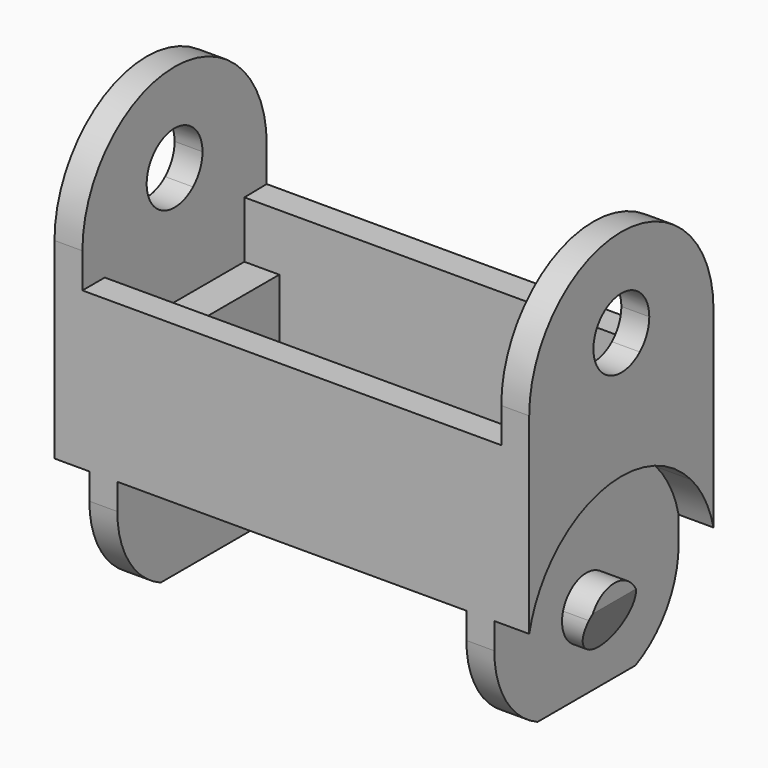
from build123d import *

# Parameters (mm, degrees)
F2_DEPTH = 1.6
F3_DEPTH = 2
F4_DEPTH = 0.4
F5_DEPTH = 11.6
F6_DEPTH = 2
F7_DEPTH = 1.6
F9_DEPTH = 25


# Not quite as in the source:
# - a feature names something its author has since deleted; it is built from what else it names


with BuildPart() as f2:
    # F1 (on offset) → F2 (new body)
    with BuildSketch(Plane.YZ.offset(11.6)):
        with BuildLine():
            Line((-0.1658547654, -17.9765316878), (-0.1658547654, -20.645576419))
            ThreePointArc((-0.1658547654, -20.645576419), (4.8341452346, -18.4390658066), (9.8341452346, -20.645576419))
            Line((9.8341452346, -20.645576419), (9.8341452346, -17.9765316878))
            Line((9.8341452346, -17.9765316878), (-0.1658547654, -17.9765316878))
        make_face()
        with BuildLine():
            Line((-0.1658547654, -23.7073743102), (-1.7658547654, -23.7073743102))
            Line((-1.7658547654, -23.7073743102), (-1.7658547654, -25.2073743102))
            Line((-1.7658547654, -25.2073743102), (-0.1658547654, -25.2073743102))
            Line((-0.1658547654, -25.2073743102), (3.1570942515, -25.2073743102))
            ThreePointArc((3.1570942515, -25.2073743102), (4.8341452346, -23.9573743102), (6.5111962178, -25.2073743102))
            Line((6.5111962178, -25.2073743102), (9.8341452346, -25.2073743102))
            Line((9.8341452346, -25.2073743102), (11.4341452346, -25.2073743102))
            Line((11.4341452346, -25.2073743102), (11.4341452346, -23.7073743102))
            Line((11.4341452346, -23.7073743102), (9.8341452346, -23.7073743102))
            Line((9.8341452346, -23.7073743102), (9.8341452346, -20.645576419))
            ThreePointArc((9.8341452346, -20.645576419), (4.8341452346, -18.4390658066), (-0.1658547654, -20.645576419))
            Line((-0.1658547654, -20.645576419), (-0.1658547654, -23.7073743102))
        make_face()
        with BuildLine():
            Line((-0.1658547654, -25.2073743102), (-1.7658547654, -25.2073743102))
            ThreePointArc((-1.7658547654, -25.2073743102), (-0.9246460766, -28.0854161792), (1.3341452346, -30.0573743102))
            Line((1.3341452346, -30.0573743102), (8.3341452346, -30.0573743102))
            ThreePointArc((8.3341452346, -30.0573743102), (10.5929365459, -28.0854161792), (11.4341452346, -25.2073743102))
            Line((11.4341452346, -25.2073743102), (9.8341452346, -25.2073743102))
            Line((9.8341452346, -25.2073743102), (6.5111962178, -25.2073743102))
            ThreePointArc((6.5111962178, -25.2073743102), (6.5658119492, -25.4547275414), (6.5841452346, -25.7073743102))
            ThreePointArc((6.5841452346, -25.7073743102), (4.5814984659, -27.4390410247), (3.1570942515, -25.2073743102))
            Line((3.1570942515, -25.2073743102), (-0.1658547654, -25.2073743102))
        make_face()
        with BuildLine():
            Line((6.5111962178, -25.2073743102), (3.1570942515, -25.2073743102))
            ThreePointArc((3.1570942515, -25.2073743102), (4.5814984659, -27.4390410247), (6.5841452346, -25.7073743102))
            ThreePointArc((6.5841452346, -25.7073743102), (6.5658119492, -25.4547275414), (6.5111962178, -25.2073743102))
        make_face()
        with BuildLine():
            ThreePointArc((6.5111962178, -25.2073743102), (4.8341452346, -23.9573743102), (3.1570942515, -25.2073743102))
            Line((3.1570942515, -25.2073743102), (6.5111962178, -25.2073743102))
        make_face()
        with BuildLine():
            Line((9.8341452346, -23.7073743102), (11.4341452346, -23.7073743102))
            ThreePointArc((11.4341452346, -23.7073743102), (10.8327827117, -22.0726736198), (9.8341452346, -20.645576419))
            Line((9.8341452346, -20.645576419), (9.8341452346, -23.7073743102))
        make_face()
        with BuildLine():
            ThreePointArc((-0.1658547654, -20.645576419), (-1.1644922425, -22.0726736198), (-1.7658547654, -23.7073743102))
            Line((-1.7658547654, -23.7073743102), (-0.1658547654, -23.7073743102))
            Line((-0.1658547654, -23.7073743102), (-0.1658547654, -20.645576419))
        make_face()
    extrude(amount=-F2_DEPTH)

    # F1 (on offset) → F3 (join)
    with BuildSketch(Plane.YZ.offset(11.6)):
        with BuildLine():
            Line((-0.1658547654, -12.7073743102), (-1.7658547654, -12.7073743102))
            Line((-1.7658547654, -12.7073743102), (-1.7658547654, -14.7073743102))
            Line((-1.7658547654, -14.7073743102), (-0.1658547654, -14.7073743102))
            Line((-0.1658547654, -14.7073743102), (-0.1658547654, -17.9765316878))
            Line((-0.1658547654, -17.9765316878), (9.8341452346, -17.9765316878))
            Line((9.8341452346, -17.9765316878), (9.8341452346, -14.7278557842))
            Line((9.8341452346, -14.7278557842), (11.4341452346, -14.7073743102))
            Line((11.4341452346, -14.7073743102), (11.4341452346, -12.7073743102))
            Line((11.4341452346, -12.7073743102), (9.8341452346, -12.7073743102))
            Line((9.8341452346, -12.7073743102), (6.1570208902, -12.7073743102))
            ThreePointArc((6.1570208902, -12.7073743102), (4.8341452346, -13.2073743102), (3.5112695791, -12.7073743102))
            Line((3.5112695791, -12.7073743102), (-0.1658547654, -12.7073743102))
        make_face()
        with BuildLine():
            ThreePointArc((11.4341452346, -12.7073743102), (4.8341452346, -6.1073743102), (-1.7658547654, -12.7073743102))
            Line((-1.7658547654, -12.7073743102), (-0.1658547654, -12.7073743102))
            Line((-0.1658547654, -12.7073743102), (3.5112695791, -12.7073743102))
            ThreePointArc((3.5112695791, -12.7073743102), (4.0112695791, -9.3844986547), (6.8341452346, -11.2073743102))
            ThreePointArc((6.8341452346, -11.2073743102), (6.6570208902, -12.0302499657), (6.1570208902, -12.7073743102))
            Line((6.1570208902, -12.7073743102), (9.8341452346, -12.7073743102))
            Line((9.8341452346, -12.7073743102), (11.4341452346, -12.7073743102))
        make_face()
        with BuildLine():
            Line((-0.1658547654, -17.9765316878), (-0.1658547654, -20.645576419))
            ThreePointArc((-0.1658547654, -20.645576419), (4.8341452346, -18.4390658066), (9.8341452346, -20.645576419))
            Line((9.8341452346, -20.645576419), (9.8341452346, -17.9765316878))
            Line((9.8341452346, -17.9765316878), (-0.1658547654, -17.9765316878))
        make_face()
    extrude(amount=F3_DEPTH)

    # F1 (on offset) → F4 (cut)
    with BuildSketch(Plane.YZ.offset(11.6)):
        with BuildLine():
            Line((-0.1658547654, -12.7073743102), (-1.7658547654, -12.7073743102))
            Line((-1.7658547654, -12.7073743102), (-1.7658547654, -14.7073743102))
            Line((-1.7658547654, -14.7073743102), (-0.1658547654, -14.7073743102))
            Line((-0.1658547654, -14.7073743102), (-0.1658547654, -17.9765316878))
            Line((-0.1658547654, -17.9765316878), (9.8341452346, -17.9765316878))
            Line((9.8341452346, -17.9765316878), (9.8341452346, -14.7278557842))
            Line((9.8341452346, -14.7278557842), (11.4341452346, -14.7073743102))
            Line((11.4341452346, -14.7073743102), (11.4341452346, -12.7073743102))
            Line((11.4341452346, -12.7073743102), (9.8341452346, -12.7073743102))
            Line((9.8341452346, -12.7073743102), (6.1570208902, -12.7073743102))
            ThreePointArc((6.1570208902, -12.7073743102), (4.8341452346, -13.2073743102), (3.5112695791, -12.7073743102))
            Line((3.5112695791, -12.7073743102), (-0.1658547654, -12.7073743102))
        make_face()
        with BuildLine():
            ThreePointArc((11.4341452346, -12.7073743102), (4.8341452346, -6.1073743102), (-1.7658547654, -12.7073743102))
            Line((-1.7658547654, -12.7073743102), (-0.1658547654, -12.7073743102))
            Line((-0.1658547654, -12.7073743102), (3.5112695791, -12.7073743102))
            ThreePointArc((3.5112695791, -12.7073743102), (4.0112695791, -9.3844986547), (6.8341452346, -11.2073743102))
            ThreePointArc((6.8341452346, -11.2073743102), (6.6570208902, -12.0302499657), (6.1570208902, -12.7073743102))
            Line((6.1570208902, -12.7073743102), (9.8341452346, -12.7073743102))
            Line((9.8341452346, -12.7073743102), (11.4341452346, -12.7073743102))
        make_face()
    extrude(amount=F4_DEPTH, mode=Mode.SUBTRACT)



with BuildPart() as f5:
    # F1 (on offset) → F5 (new body)
    with BuildSketch(Plane.YZ.offset(11.6)):
        with BuildLine():
            Line((11.4341452346, -23.7073743102), (11.4341452346, -14.7073743102))
            Line((11.4341452346, -14.7073743102), (9.8341452346, -14.7278557842))
            Line((9.8341452346, -14.7278557842), (9.8341452346, -17.9765316878))
            Line((9.8341452346, -17.9765316878), (9.8341452346, -20.645576419))
            ThreePointArc((9.8341452346, -20.645576419), (10.8327827117, -22.0726736198), (11.4341452346, -23.7073743102))
        make_face()
        with BuildLine():
            Line((9.8341452346, -23.7073743102), (11.4341452346, -23.7073743102))
            ThreePointArc((11.4341452346, -23.7073743102), (10.8327827117, -22.0726736198), (9.8341452346, -20.645576419))
            Line((9.8341452346, -20.645576419), (9.8341452346, -23.7073743102))
        make_face()
    extrude(amount=-F5_DEPTH)


with BuildPart() as f5b:
    # F1 (on offset) → F5, piece 2 (new body)
    with BuildSketch(Plane.YZ.offset(11.6)):
        with BuildLine():
            Line((-0.1658547654, -14.7073743102), (-1.7658547654, -14.7073743102))
            Line((-1.7658547654, -14.7073743102), (-1.7658547654, -23.7073743102))
            ThreePointArc((-1.7658547654, -23.7073743102), (-1.1644922425, -22.0726736198), (-0.1658547654, -20.645576419))
            Line((-0.1658547654, -20.645576419), (-0.1658547654, -17.9765316878))
            Line((-0.1658547654, -17.9765316878), (-0.1658547654, -14.7073743102))
        make_face()
        with BuildLine():
            ThreePointArc((-0.1658547654, -20.645576419), (-1.1644922425, -22.0726736198), (-1.7658547654, -23.7073743102))
            Line((-1.7658547654, -23.7073743102), (-0.1658547654, -23.7073743102))
            Line((-0.1658547654, -23.7073743102), (-0.1658547654, -20.645576419))
        make_face()
    extrude(amount=-F5_DEPTH)


with BuildPart() as f2_1:
    add(f2.part)

    add(f5.part)  # F6 merges F5

    add(f5b.part)  # F6 merges F5b
    # F1 (on offset) → F6 (join)
    with BuildSketch(Plane.YZ.offset(11.6)):
        with BuildLine():
            Line((-0.1658547654, -14.7073743102), (-1.7658547654, -14.7073743102))
            Line((-1.7658547654, -14.7073743102), (-1.7658547654, -23.7073743102))
            ThreePointArc((-1.7658547654, -23.7073743102), (-1.1644922425, -22.0726736198), (-0.1658547654, -20.645576419))
            Line((-0.1658547654, -20.645576419), (-0.1658547654, -17.9765316878))
            Line((-0.1658547654, -17.9765316878), (-0.1658547654, -14.7073743102))
        make_face()
        with BuildLine():
            Line((11.4341452346, -23.7073743102), (11.4341452346, -14.7073743102))
            Line((11.4341452346, -14.7073743102), (9.8341452346, -14.7278557842))
            Line((9.8341452346, -14.7278557842), (9.8341452346, -17.9765316878))
            Line((9.8341452346, -17.9765316878), (9.8341452346, -20.645576419))
            ThreePointArc((9.8341452346, -20.645576419), (10.8327827117, -22.0726736198), (11.4341452346, -23.7073743102))
        make_face()
    extrude(amount=F6_DEPTH)

    # F1 (on offset) → F7 (join)
    with BuildSketch(Plane.YZ.offset(11.6)):
        with BuildLine():
            ThreePointArc((6.5111962178, -25.2073743102), (4.8341452346, -23.9573743102), (3.1570942515, -25.2073743102))
            Line((3.1570942515, -25.2073743102), (6.5111962178, -25.2073743102))
        make_face()
        with BuildLine():
            Line((6.5111962178, -25.2073743102), (3.1570942515, -25.2073743102))
            ThreePointArc((3.1570942515, -25.2073743102), (4.5814984659, -27.4390410247), (6.5841452346, -25.7073743102))
            ThreePointArc((6.5841452346, -25.7073743102), (6.5658119492, -25.4547275414), (6.5111962178, -25.2073743102))
        make_face()
    extrude(amount=F7_DEPTH)

    # F8 (on Front) → F9 (cut)
    with BuildSketch(Plane.XZ):
        Polygon((14.5103234728, -25.0094107672), (13.301373871, -24.5876735715), (12.2712288238, -27.5406818837), (13.4801784256, -27.9624190794), align=None)
    extrude(amount=-F9_DEPTH, mode=Mode.SUBTRACT)

    # F10: F2 across plane


with BuildPart() as f2_2:
    add(f2_1.part)
    add(f2_1.part.mirror(Plane.YZ))


with BuildPart() as f11_1:
    # F11: copy of F2
    add(f2_2.part)


solid = f2_2.part
